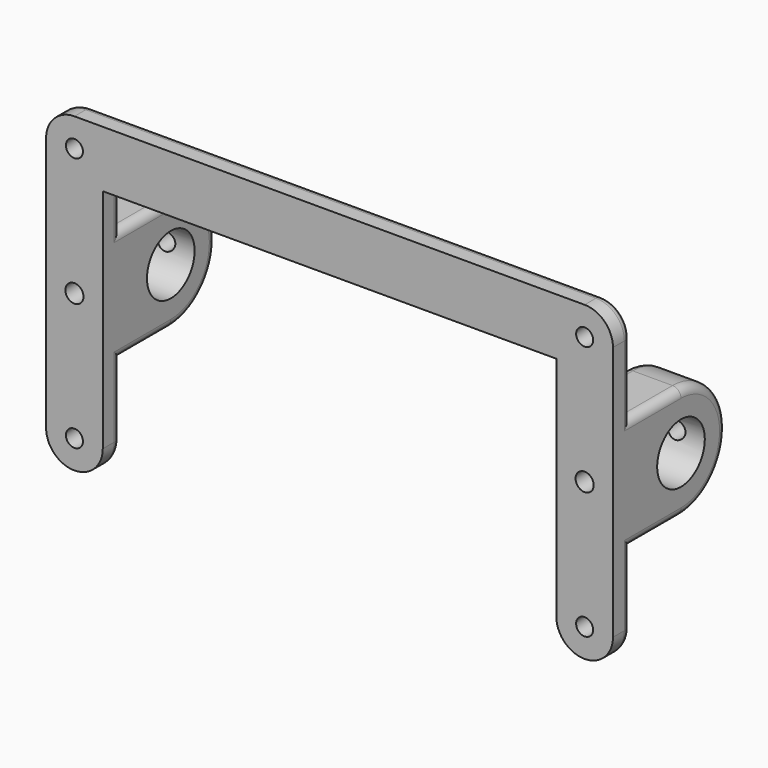
from build123d import *

# Parameters (mm, degrees)
F0_W      = 5
F0_H      = 10
F0_H_2    = 5
F0_W_2    = 80
F0_H_3    = 35
F1_DEPTH  = 4
F3_D      = 3
F4_W      = 10
F4_H      = 10
F5_DEPTH  = 25
F7_D      = 10.5
F7_DEPTH  = 10.001
F9_D      = 10.5
F10_R     = 9.99999
F11_R     = 4.99999
F13_D     = 3.2
F13_DEPTH = 25
F13_TIP   = 0.9613769904
F14_R     = 1.5


# Not quite as in the source:
# - a fillet or chamfer is up to 0.001 mm smaller than in the source, because OpenCascade refuses the exact size
# - a feature names something its author has since deleted; it is built from what else it names


with BuildPart() as f1:
    # F0 (on Front) → F1 (new body)
    with BuildSketch(Plane.XZ):
        with Locations((-82.5, 50)):
            Rectangle(F0_W, F0_H)
        with Locations((-87.5, 50)):
            Rectangle(F0_W, F0_H)
        with Locations((-87.5, 5)):
            Rectangle(F0_W, F0_H)
        with Locations((-82.5, 5)):
            Rectangle(F0_W, F0_H)
        with Locations((2.5, 50)):
            Rectangle(F0_W, F0_H)
        with Locations((7.5, 50)):
            Rectangle(F0_W, F0_H)
        with Locations((2.5, 7.5)):
            Rectangle(F0_W, F0_H_2)
        with Locations((7.5, 7.5)):
            Rectangle(F0_W, F0_H_2)
        with Locations((7.5, 2.5)):
            Rectangle(F0_W, F0_H_2)
        with Locations((2.5, 2.5)):
            Rectangle(F0_W, F0_H_2)
        with Locations((-40, 50)):
            Rectangle(F0_W_2, F0_H)
        with Locations((2.5, 27.5)):
            Rectangle(F0_W, F0_H_3)
        with Locations((7.5, 27.5)):
            Rectangle(F0_W, F0_H_3)
        with Locations((-82.5, 27.5)):
            Rectangle(F0_W, F0_H_3)
        with Locations((-87.5, 27.5)):
            Rectangle(F0_W, F0_H_3)
    extrude(amount=-F1_DEPTH)

    # F3 (through all)
    with Locations(Plane.XZ):
        with Locations((5, 50), (-85, 50), (5, 5), (-85, 5)):
            Hole(F3_D / 2)

    # F4 (on Front) → F5 (join)
    with BuildSketch(Plane.XZ):
        with Locations((5, 22.5)):
            Rectangle(F4_W, F4_H)
        with Locations((5, 32.5)):
            Rectangle(F4_W, F4_H)
        with Locations((-85, 22.5)):
            Rectangle(F4_W, F4_H)
        with Locations((-85, 32.5)):
            Rectangle(F4_W, F4_H)
    extrude(amount=-F5_DEPTH)

    # F7 (through all, one way)
    with BuildSketch(Plane(origin=(0, 0, 0), x_dir=(0, 1, 0), z_dir=(-1, 0, 0))):
        with Locations((15, -27.5)):
            Circle(F7_D / 2)
    extrude(amount=-F7_DEPTH, mode=Mode.SUBTRACT)

    # F9 (through all)
    with Locations(Plane.YZ):
        with Locations((15, 27.5)):
            Hole(F9_D / 2)

    # F10 (radius 10 in the source; OpenCascade refuses exactly that, so slightly less here)
    f10_edges = [f1.edges().sort_by_distance(p)[0] for p in [
        (5, 25, 37.5),
        (5, 25, 17.5),
        (-85, 25, 37.5),
        (-85, 25, 17.5),
    ]]
    fillet(f10_edges, radius=F10_R)

    # F11 (radius 5 in the source; OpenCascade refuses exactly that, so slightly less here)
    f11_edges = [f1.edges().sort_by_distance(p)[0] for p in [
        (10, 2, 0),
        (-90, 2, 0),
        (-80, 2, 0),
        (-90, 2, 55),
        (10, 2, 55),
        (0, 2, 0),
    ]]
    fillet(f11_edges, radius=F11_R)

    # F13
    with Locations(Plane.XZ):
        with Locations((5, 27.5), (-85, 27.5)):
            Hole(F13_D / 2, depth=F13_DEPTH)
            with Locations((0, 0, -(F13_DEPTH + F13_TIP / 2))):  # 118° drill point
                Cone(0, F13_D / 2, F13_TIP, mode=Mode.SUBTRACT)

    # F14
    f14_edges = [f1.edges().sort_by_distance(p)[0] for p in [
        (-40, 4, 55),
        (10, 22.071071, 34.571071),
        (10, 4, 11.249995),
        (0, 22.071071, 34.571071),
        (0, 4, 41.25),
        (-40, 4, 45),
        (-80, 4, 41.25),
        (-80, 22.071071, 34.571071),
        (-90, 22.071071, 34.571071),
        (-90, 4, 11.249995),
    ]]
    fillet(f14_edges, radius=F14_R)


solid = f1.part
